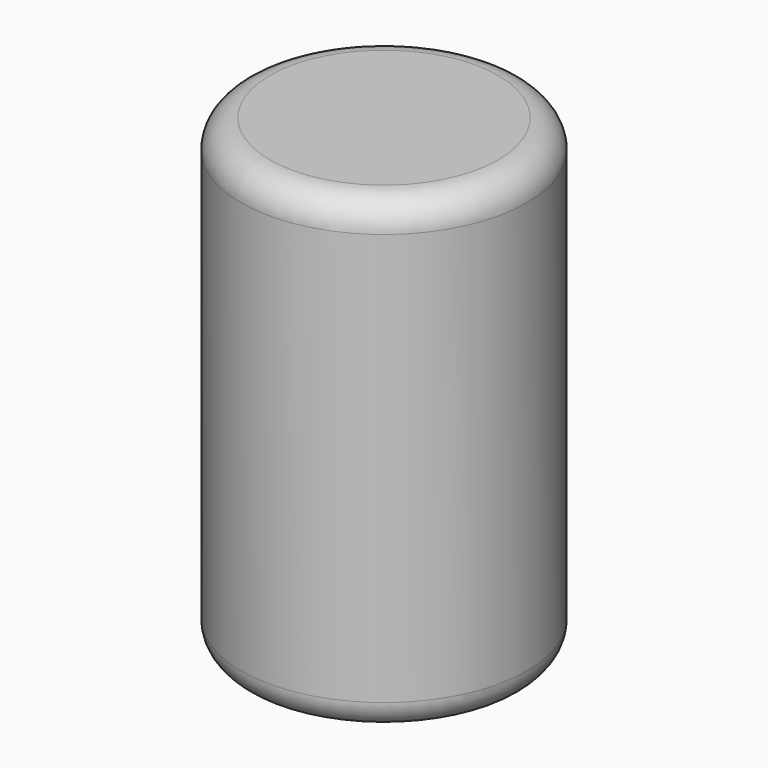
from build123d import *

# Parameters (mm, degrees)
F0_R     = 38.1
F1_DEPTH = 123.825
F2_R     = 34.925
F3_DEPTH = 111.125
F5_R     = 7.62


# Not quite as in the source:
# - a fillet or chamfer that OpenCascade refuses, or shapes differently, is made with other operations: its cross-section is extruded or revolved along the edge and cut away or added


with BuildPart() as f1:
    # F0 (on Top) → F1 (new body)
    with BuildSketch(Plane.XY):
        Circle(F0_R)
    extrude(amount=F1_DEPTH)

    # F2 (on Top) → F3 (cut)
    with BuildSketch(Plane.XY):
        Circle(F2_R)
    extrude(amount=F3_DEPTH, mode=Mode.SUBTRACT)

    # F4: fillet of radius 7.62 on 1 edges, made by hand

    # F4_s1 → F4_t2 (revolve, cut)
    with BuildSketch(Plane.XZ):
        with BuildLine():
            ThreePointArc((38.1, 6.189214409), (37.25994469, 2.7111761688), (34.925, 0))
            Line((34.925, 0), (38.1, 0))
            Line((38.1, 0), (38.1, 6.189214409))
        make_face()
    revolve(axis=Axis((0, 0, 0), (0, 0, 1)), mode=Mode.SUBTRACT)

    # F5
    f5_edges = [f1.edges().sort_by_distance(p)[0] for p in [
        (-38.1, 0, 123.825),
    ]]
    fillet(f5_edges, radius=F5_R)


solid = f1.part
